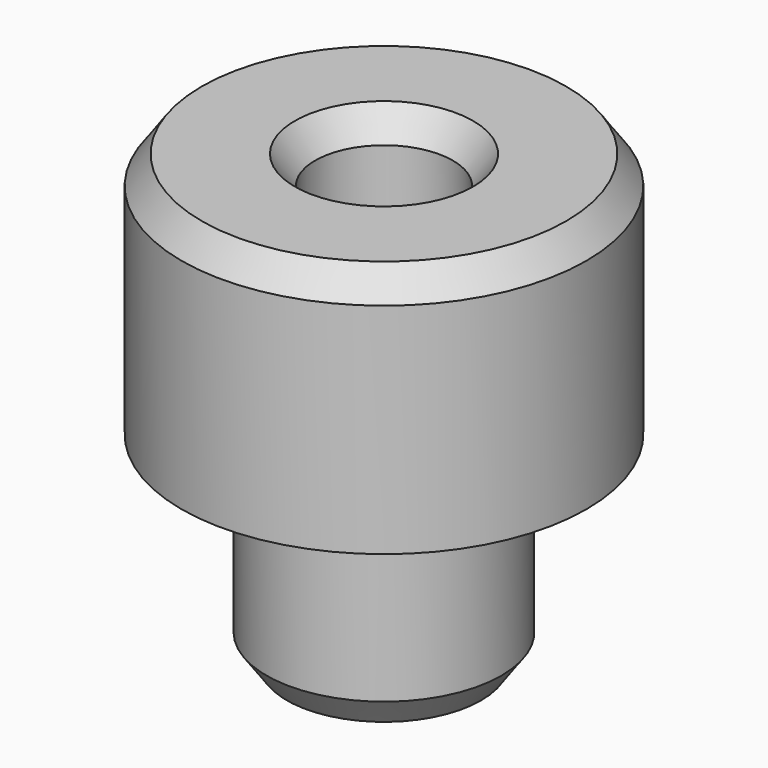
from build123d import *

# Parameters (mm, degrees)
F2_C1_SIZE2 = 0.5
F2_C1_SIZE  = 0.7
F2_C2_SIZE2 = 0.7
F2_C2_SIZE  = 0.5
F2_C3_SIZE2 = 0.7
F2_C3_SIZE  = 0.5


with BuildPart() as f1:
    # F0 (on Front) → F1 (revolve)
    with BuildSketch(Plane.XZ):
        Polygon((0.7, 6), (0.7, 0), (2.9, 0), (2.9, 5.4), (3.65, 5.4), (3.65, 5), (5, 5), (5, 11.1), (1.7, 11.1), (1.7, 6), align=None)
    revolve(axis=Axis((0, 0, 5.55), (0, 0, -1)))

    # F2: chamfer of 0.7 x 0.5 on 3 edges, made by hand

    # F2_c1
    f2_c1_edges = [f1.edges().sort_by_distance(p)[0] for p in [
        (-1.7, 0, 11.1),
    ]]
    f2_c1_side = f1.faces().sort_by_distance((-1.7, 0, 11.09))[0]
    chamfer(f2_c1_edges, length=F2_C1_SIZE, length2=F2_C1_SIZE2, reference=f2_c1_side)

    # F2_c2
    f2_c2_edges = [f1.edges().sort_by_distance(p)[0] for p in [
        (-2.9, 0, 0),
    ]]
    f2_c2_side = f1.faces().sort_by_distance((-2.89, 0, 0))[0]
    chamfer(f2_c2_edges, length=F2_C2_SIZE, length2=F2_C2_SIZE2, reference=f2_c2_side)

    # F2_c3
    f2_c3_edges = [f1.edges().sort_by_distance(p)[0] for p in [
        (-5, 0, 11.1),
    ]]
    f2_c3_side = f1.faces().sort_by_distance((-4.99, 0, 11.1))[0]
    chamfer(f2_c3_edges, length=F2_C3_SIZE, length2=F2_C3_SIZE2, reference=f2_c3_side)


solid = f1.part
